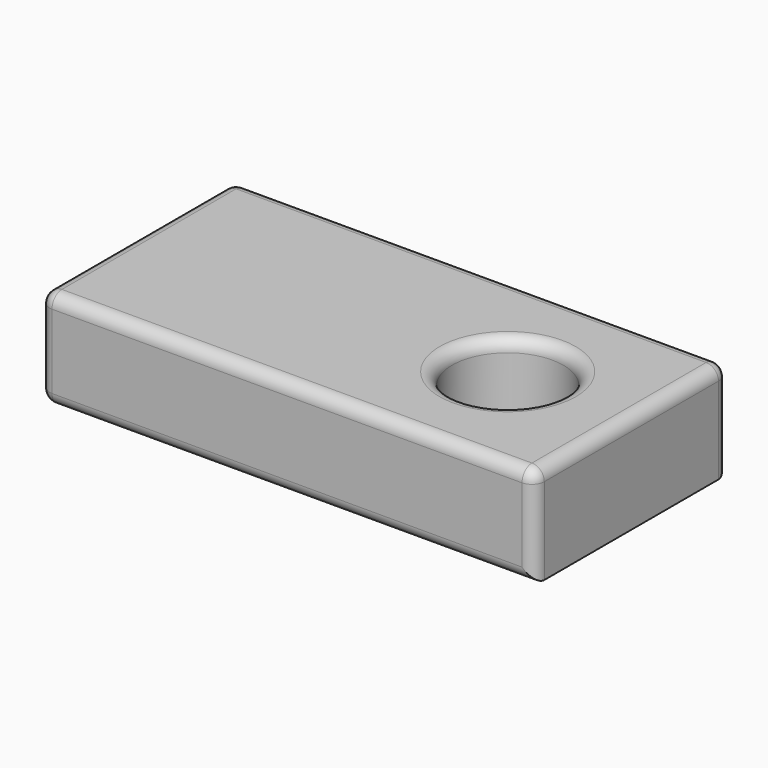
from build123d import *

# Parameters (mm, degrees)
F0_R         = 2.25
F1_DEPTH     = 4
F2_W         = 9
F2_H         = 3
F3_DEPTH     = 2
F4_R         = 0.5
F5_T1_DEPTH  = 8.5
F5_T3_DEPTH  = 2
F5_T5_DEPTH  = 2.9
F5_T7_DEPTH  = 2.9
F5_S11_W     = 0.5
F5_S11_H     = 0.5
F5_T12_DEPTH = 0.5
F5_S17_W     = 0.5
F5_S17_H     = 0.5
F5_T18_DEPTH = 0.5
F5_T22_ANGLE = 90
F5_T24_ANGLE = 90
F5_T29_DEPTH = 9.75
F5_T33_DEPTH = 3.25
F5_T40_DEPTH = 9.75
F5_T44_DEPTH = 3.25


# Not quite as in the source:
# - a fillet or chamfer that OpenCascade refuses, or shapes differently, is made with other operations: its cross-section is extruded or revolved along the edge and cut away or added


with BuildPart() as f1:
    # F0 (on Top) → F1 (new body)
    with BuildSketch(Plane.XY):
        with BuildLine():
            Line((20, 0), (20, 9.8))
            Line((20, 9.8), (0, 9.8))
            Line((0, 9.8), (0, 6.4))
            ThreePointArc((0, 6.4), (0.1464466094, 6.0464466094), (0.5, 5.9))
            Line((0.5, 5.9), (9, 5.9))
            Line((9, 5.9), (9, 3.9))
            Line((9, 3.9), (0.5, 3.9))
            ThreePointArc((0.5, 3.9), (0.1464466094, 3.7535533906), (0, 3.4))
            Line((0, 3.4), (0, 0))
            Line((0, 0), (20, 0))
        make_face()
        with Locations((15, 4.9)):
            Circle(F0_R, mode=Mode.SUBTRACT)
    extrude(amount=F1_DEPTH)

    # F2 (on face) → F3 (join)
    with BuildSketch(Plane.XY.offset(4)):
        with Locations((4.5, 4.9)):
            Rectangle(F2_W, F2_H)
    extrude(amount=-F3_DEPTH)

    # F4
    f4_edges = [f1.edges().sort_by_distance(p)[0] for p in [
        (10, 0, 4),
        (20, 4.9, 4),
        (10, 9.8, 4),
        (0, 4.9, 4),
        (12.75, 4.9, 4),
        (20, 9.8, 2),
        (0, 9.8, 2),
        (10, 9.8, 0),
        (0, 0, 2),
        (20, 0, 2),
        (10, 0, 0),
    ]]
    fillet(f4_edges, radius=F4_R)

    # F5: fillet of radius 0.5 on 3 edges, made by hand

    # F5_s2 → F5_t1 (cut)
    with BuildSketch(Plane.YZ.offset(0.5)):
        with BuildLine():
            ThreePointArc((6.4, 0), (6.0464466094, 0.1464466094), (5.9, 0.5))
            Line((5.9, 0.5), (5.9, 0))
            Line((5.9, 0), (6.4, 0))
        make_face()
        with BuildLine():
            ThreePointArc((3.4, 0), (3.7535533906, 0.1464466094), (3.9, 0.5))
            Line((3.9, 0.5), (3.9, 0))
            Line((3.9, 0), (3.4, 0))
        make_face()
    extrude(amount=F5_T1_DEPTH, mode=Mode.SUBTRACT)

    # F5_s4 → F5_t3 (cut)
    with BuildSketch(Plane.XZ.offset(-5.9)):
        with BuildLine():
            ThreePointArc((9.5, 0), (9.1464466094, 0.1464466094), (9, 0.5))
            Line((9, 0.5), (9, 0))
            Line((9, 0), (9.5, 0))
        make_face()
    extrude(amount=F5_T3_DEPTH, mode=Mode.SUBTRACT)

    # F5_s6 → F5_t5 (cut)
    with BuildSketch(Plane.XZ.offset(-3.4)):
        with BuildLine():
            ThreePointArc((0.5, 0), (0.1464466094, 0.1464466094), (0, 0.5))
            Line((0, 0.5), (0, 0))
            Line((0, 0), (0.5, 0))
        make_face()
    extrude(amount=F5_T5_DEPTH, mode=Mode.SUBTRACT)

    # F5_s8 → F5_t7 (cut)
    with BuildSketch(Plane.XZ.offset(-9.3)):
        with BuildLine():
            ThreePointArc((0.5, 0), (0.1464466094, 0.1464466094), (0, 0.5))
            Line((0, 0.5), (0, 0))
            Line((0, 0), (0.5, 0))
        make_face()
    extrude(amount=F5_T7_DEPTH, mode=Mode.SUBTRACT)


with BuildPart() as f5_tool10:
    # F5_s11 → F5_t12 (new body)
    with BuildSketch(Plane.XY.offset(0.5)):
        with Locations((0.25, 0.25)):
            Rectangle(F5_S11_W, F5_S11_H)
    extrude(amount=-F5_T12_DEPTH)

    # F5_s13 → F5_t14 (revolve, cut)
    with BuildSketch(Plane(origin=(0.5, 0.5, 0.5), x_dir=(0.7071067812, 0.7071067812, 0), z_dir=(-0.7071067812, 0.7071067812, 0))):
        with BuildLine():
            ThreePointArc((0, -0.5), (0.5, 0), (0, 0.5))
            Line((0, 0.5), (0, -0.5))
        make_face()
    revolve(axis=Axis((0.5, 0.5, 0.5), (0, 0, -1)), mode=Mode.SUBTRACT)


with BuildPart() as f1_1:
    add(f1.part)

    # F5_t9: cut F5_tool10
    add(f5_tool10.part, mode=Mode.SUBTRACT)


with BuildPart() as f5_tool16:
    # F5_s17 → F5_t18 (new body)
    with BuildSketch(Plane.XY.offset(0.5)):
        with Locations((0.25, 9.55)):
            Rectangle(F5_S17_W, F5_S17_H)
    extrude(amount=-F5_T18_DEPTH)

    # F5_s19 → F5_t20 (revolve, cut)
    with BuildSketch(Plane(origin=(0.5, 9.3, 0.5), x_dir=(0.7071067812, -0.7071067812, 0), z_dir=(0.7071067812, 0.7071067812, 0))):
        with BuildLine():
            ThreePointArc((0, -0.5), (0.5, 0), (0, 0.5))
            Line((0, 0.5), (0, -0.5))
        make_face()
    revolve(axis=Axis((0.5, 9.3, 0.5), (0, 0, -1)), mode=Mode.SUBTRACT)


with BuildPart() as f1_2:
    add(f1_1.part)

    # F5_t15: cut F5_tool16
    add(f5_tool16.part, mode=Mode.SUBTRACT)

    # F5_s21 → F5_t22 (revolve, cut)
    with BuildSketch(Plane.YZ.offset(0.5)):
        with BuildLine():
            ThreePointArc((3.4, 0), (3.7535533906, 0.1464466094), (3.9, 0.5))
            Line((3.9, 0.5), (3.9, 0))
            Line((3.9, 0), (3.4, 0))
        make_face()
    revolve(axis=Axis((0.5, 3.4, 0), (0, 0, 1)), revolution_arc=F5_T22_ANGLE, mode=Mode.SUBTRACT)

    # F5_s23 → F5_t24 (revolve, cut)
    with BuildSketch(Plane.XZ.offset(-6.4)):
        with BuildLine():
            ThreePointArc((0.5, 0), (0.1464466094, 0.1464466094), (0, 0.5))
            Line((0, 0.5), (0, 0))
            Line((0, 0), (0.5, 0))
        make_face()
    revolve(axis=Axis((0.5, 6.4, 0), (0, 0, 1)), revolution_arc=F5_T24_ANGLE, mode=Mode.SUBTRACT)


with BuildPart() as f5_tool27:
    # F5_s28 → F5_t29 (new body)
    with BuildSketch(Plane.YZ.offset(0.5)):
        with BuildLine():
            ThreePointArc((6.4, 0), (6.0464466094, 0.1464466094), (5.9, 0.5))
            Line((5.9, 0.5), (5.9, 0))
            Line((5.9, 0), (6.4, 0))
        make_face()
    extrude(amount=F5_T29_DEPTH)

    split(bisect_by=Plane.YZ.offset(9), keep=Keep.TOP)


with BuildPart() as f5_tool31:
    # F5_s32 → F5_t33 (new body)
    with BuildSketch(Plane.XZ.offset(-7.15)):
        with BuildLine():
            ThreePointArc((9.5, 0), (9.1464466094, 0.1464466094), (9, 0.5))
            Line((9, 0.5), (9, 0))
            Line((9, 0), (9.5, 0))
        make_face()
    extrude(amount=F5_T33_DEPTH)

    split(bisect_by=Plane.XZ.offset(-5.9), keep=Keep.BOTTOM)


with BuildPart() as f5_tool27_1:
    add(f5_tool27.part)

    # F5_t35: intersect F5_tool31
    add(f5_tool31.part, mode=Mode.INTERSECT)


with BuildPart() as f1_3:
    add(f1_2.part)

    # F5_t25: cut F5_tool27
    add(f5_tool27_1.part, mode=Mode.SUBTRACT)


with BuildPart() as f5_tool38:
    # F5_s39 → F5_t40 (new body)
    with BuildSketch(Plane.YZ.offset(10.25)):
        with BuildLine():
            ThreePointArc((3.4, 0), (3.7535533906, 0.1464466094), (3.9, 0.5))
            Line((3.9, 0.5), (3.9, 0))
            Line((3.9, 0), (3.4, 0))
        make_face()
    extrude(amount=-F5_T40_DEPTH)

    split(bisect_by=Plane.YZ.offset(9), keep=Keep.TOP)


with BuildPart() as f5_tool42:
    # F5_s43 → F5_t44 (new body)
    with BuildSketch(Plane.XZ.offset(-5.9)):
        with BuildLine():
            ThreePointArc((9.5, 0), (9.1464466094, 0.1464466094), (9, 0.5))
            Line((9, 0.5), (9, 0))
            Line((9, 0), (9.5, 0))
        make_face()
    extrude(amount=F5_T44_DEPTH)

    split(bisect_by=Plane.XZ.offset(-3.9), keep=Keep.TOP)


with BuildPart() as f5_tool38_1:
    add(f5_tool38.part)

    # F5_t46: intersect F5_tool42
    add(f5_tool42.part, mode=Mode.INTERSECT)


with BuildPart() as f1_4:
    add(f1_3.part)

    # F5_t36: cut F5_tool38
    add(f5_tool38_1.part, mode=Mode.SUBTRACT)


solid = f1_4.part
